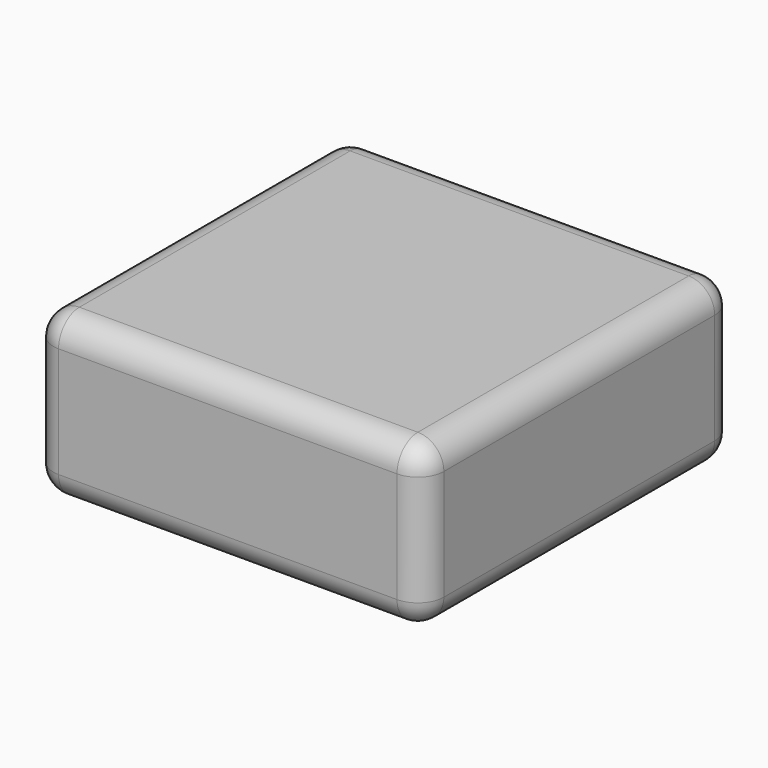
from build123d import *

# Parameters (mm, degrees)
F0_W         = 76.2
F0_H         = 76.2
F1_DEPTH     = 31.75
F2_R         = 5.08
F3_T1_DEPTH  = 66.04
F3_T3_DEPTH  = 21.59
F3_T5_DEPTH  = 66.04
F3_S9_W      = 5.08
F3_S9_H      = 5.08
F3_T10_DEPTH = 5.08
F3_S15_W     = 5.08
F3_S15_H     = 5.08
F3_T16_DEPTH = 5.08
F3_S21_W     = 5.08
F3_S21_H     = 5.08
F3_T22_DEPTH = 5.08
F3_S27_W     = 5.08
F3_S27_H     = 5.08
F3_T28_DEPTH = 5.08
F3_T32_ANGLE = 90


# Not quite as in the source:
# - a fillet or chamfer that OpenCascade refuses, or shapes differently, is made with other operations: its cross-section is extruded or revolved along the edge and cut away or added


with BuildPart() as f1:
    # F0 (on Top) → F1 (new body)
    with BuildSketch(Plane.XY):
        Rectangle(F0_W, F0_H)
    extrude(amount=-F1_DEPTH)

    # F2
    f2_edges = [f1.edges().sort_by_distance(p)[0] for p in [
        (0, -38.1, 0),
        (38.1, -38.1, -15.875),
        (38.1, 0, 0),
        (38.1, 38.1, -15.875),
        (38.1, 0, -31.75),
        (0, -38.1, -31.75),
        (-38.1, 0, 0),
        (0, 38.1, 0),
    ]]
    fillet(f2_edges, radius=F2_R)

    # F3: fillet of radius 5.08 on 5 edges, made by hand

    # F3_s2 → F3_t1 (cut)
    with BuildSketch(Plane.YZ.offset(-33.02)):
        with BuildLine():
            ThreePointArc((33.02, -31.75), (36.6121024484, -30.2621024484), (38.1, -26.67))
            Line((38.1, -26.67), (38.1, -31.75))
            Line((38.1, -31.75), (33.02, -31.75))
        make_face()
    extrude(amount=F3_T1_DEPTH, mode=Mode.SUBTRACT)

    # F3_s4 → F3_t3 (cut)
    with BuildSketch(Plane.XY.offset(-26.67)):
        with BuildLine():
            ThreePointArc((-33.02, 38.1), (-36.6121024484, 36.6121024484), (-38.1, 33.02))
            Line((-38.1, 33.02), (-38.1, 38.1))
            Line((-38.1, 38.1), (-33.02, 38.1))
        make_face()
        with BuildLine():
            ThreePointArc((-33.02, -38.1), (-36.6121024484, -36.6121024484), (-38.1, -33.02))
            Line((-38.1, -33.02), (-38.1, -38.1))
            Line((-38.1, -38.1), (-33.02, -38.1))
        make_face()
    extrude(amount=F3_T3_DEPTH, mode=Mode.SUBTRACT)

    # F3_s6 → F3_t5 (cut)
    with BuildSketch(Plane.XZ.offset(-33.02)):
        with BuildLine():
            ThreePointArc((-33.02, -31.75), (-36.6121024484, -30.2621024484), (-38.1, -26.67))
            Line((-38.1, -26.67), (-38.1, -31.75))
            Line((-38.1, -31.75), (-33.02, -31.75))
        make_face()
    extrude(amount=F3_T5_DEPTH, mode=Mode.SUBTRACT)


with BuildPart() as f3_tool8:
    # F3_s9 → F3_t10 (new body)
    with BuildSketch(Plane.XZ.offset(33.02)):
        with Locations((-35.56, -2.54)):
            Rectangle(F3_S9_W, F3_S9_H)
    extrude(amount=F3_T10_DEPTH)

    # F3_s11 → F3_t12 (revolve, cut)
    with BuildSketch(Plane(origin=(-33.02, -33.02, -5.08), x_dir=(0.7071067812, 0, -0.7071067812), z_dir=(-0.7071067812, 0, -0.7071067812))):
        with BuildLine():
            ThreePointArc((0, -5.08), (5.08, 0), (0, 5.08))
            Line((0, 5.08), (0, -5.08))
        make_face()
    revolve(axis=Axis((-33.02, -33.02, -5.08), (0, -1, 0)), mode=Mode.SUBTRACT)


with BuildPart() as f1_1:
    add(f1.part)

    # F3_t7: cut F3_tool8
    add(f3_tool8.part, mode=Mode.SUBTRACT)


with BuildPart() as f3_tool14:
    # F3_s15 → F3_t16 (new body)
    with BuildSketch(Plane.XZ.offset(-33.02)):
        with Locations((-35.56, -2.54)):
            Rectangle(F3_S15_W, F3_S15_H)
    extrude(amount=-F3_T16_DEPTH)

    # F3_s17 → F3_t18 (revolve, cut)
    with BuildSketch(Plane(origin=(-33.02, 33.02, -5.08), x_dir=(0.7071067812, 0, -0.7071067812), z_dir=(0.7071067812, 0, 0.7071067812))):
        with BuildLine():
            ThreePointArc((0, -5.08), (5.08, 0), (0, 5.08))
            Line((0, 5.08), (0, -5.08))
        make_face()
    revolve(axis=Axis((-33.02, 33.02, -5.08), (0, 1, 0)), mode=Mode.SUBTRACT)


with BuildPart() as f1_2:
    add(f1_1.part)

    # F3_t13: cut F3_tool14
    add(f3_tool14.part, mode=Mode.SUBTRACT)


with BuildPart() as f3_tool20:
    # F3_s21 → F3_t22 (new body)
    with BuildSketch(Plane.XY.offset(-26.67)):
        with Locations((35.56, 35.56)):
            Rectangle(F3_S21_W, F3_S21_H)
    extrude(amount=-F3_T22_DEPTH)

    # F3_s23 → F3_t24 (revolve, cut)
    with BuildSketch(Plane(origin=(33.02, 33.02, -26.67), x_dir=(-0.7071067812, -0.7071067812, 0), z_dir=(0.7071067812, -0.7071067812, 0))):
        with BuildLine():
            ThreePointArc((0, -5.08), (5.08, 0), (0, 5.08))
            Line((0, 5.08), (0, -5.08))
        make_face()
    revolve(axis=Axis((33.02, 33.02, -26.67), (0, 0, -1)), mode=Mode.SUBTRACT)


with BuildPart() as f1_3:
    add(f1_2.part)

    # F3_t19: cut F3_tool20
    add(f3_tool20.part, mode=Mode.SUBTRACT)


with BuildPart() as f3_tool26:
    # F3_s27 → F3_t28 (new body)
    with BuildSketch(Plane.XY.offset(-26.67)):
        with Locations((-35.56, 35.56)):
            Rectangle(F3_S27_W, F3_S27_H)
    extrude(amount=-F3_T28_DEPTH)

    # F3_s29 → F3_t30 (revolve, cut)
    with BuildSketch(Plane(origin=(-33.02, 33.02, -26.67), x_dir=(0.7071067812, -0.7071067812, 0), z_dir=(0.7071067812, 0.7071067812, 0))):
        with BuildLine():
            ThreePointArc((0, -5.08), (5.08, 0), (0, 5.08))
            Line((0, 5.08), (0, -5.08))
        make_face()
    revolve(axis=Axis((-33.02, 33.02, -26.67), (0, 0, -1)), mode=Mode.SUBTRACT)


with BuildPart() as f1_4:
    add(f1_3.part)

    # F3_t25: cut F3_tool26
    add(f3_tool26.part, mode=Mode.SUBTRACT)

    # F3_s31 → F3_t32 (revolve, cut)
    with BuildSketch(Plane.XY.offset(-26.67)):
        with BuildLine():
            ThreePointArc((-38.1, -33.02), (-36.6121024484, -36.6121024484), (-33.02, -38.1))
            Line((-33.02, -38.1), (-38.1, -38.1))
            Line((-38.1, -38.1), (-38.1, -33.02))
        make_face()
    revolve(axis=Axis((-38.1, -33.02, -26.67), (1, 0, 0)), revolution_arc=F3_T32_ANGLE, mode=Mode.SUBTRACT)


solid = f1_4.part
